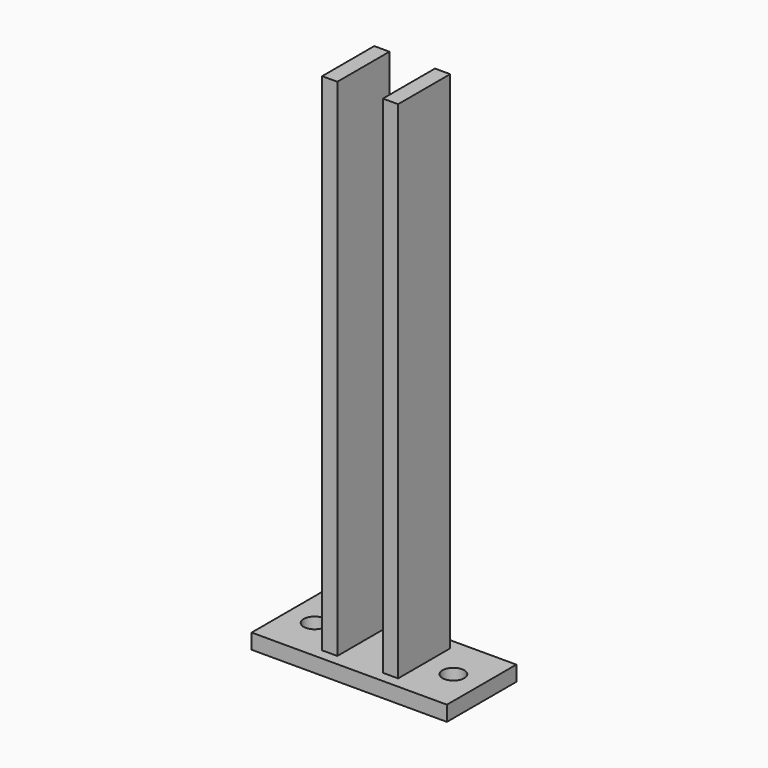
from build123d import *

# Parameters (mm, degrees)
F0_W     = 40
F0_H     = 7
F1_DEPTH = 90
F4_D     = 10
F5_W     = 7
F5_H     = 240
F6_DEPTH = 15
F7_DEPTH = 15


# Not quite as in the source:
# - a feature names something its author has since deleted; it is built from what else it names


with BuildPart() as f1:
    # F0 (on Right) → F1 (new body)
    with BuildSketch(Plane.YZ):
        with Locations((0, 3.5)):
            Rectangle(F0_W, F0_H)
    extrude(amount=F1_DEPTH)

    # F4 (through all)
    with Locations(Plane(origin=(0, 0, 0), x_dir=(1, 0, 0), z_dir=(0, 0, -1))):
        with Locations((13, 0), (77, 0)):
            Hole(F4_D / 2)

    # F5 (on Front) → F6 (join)
    with BuildSketch(Plane.XZ):
        with Locations((60, 120)):
            Rectangle(F5_W, F5_H)
        with Locations((32, 120)):
            Rectangle(F5_W, F5_H)
    extrude(amount=F6_DEPTH)

    # F7 (add): faces of the model
    f7_faces = [f1.faces().sort_by_distance(p)[0] for p in [
        (32, 0, 123.5),
        (60, 0, 123.5),
    ]]
    extrude(f7_faces, amount=F7_DEPTH)


solid = f1.part
